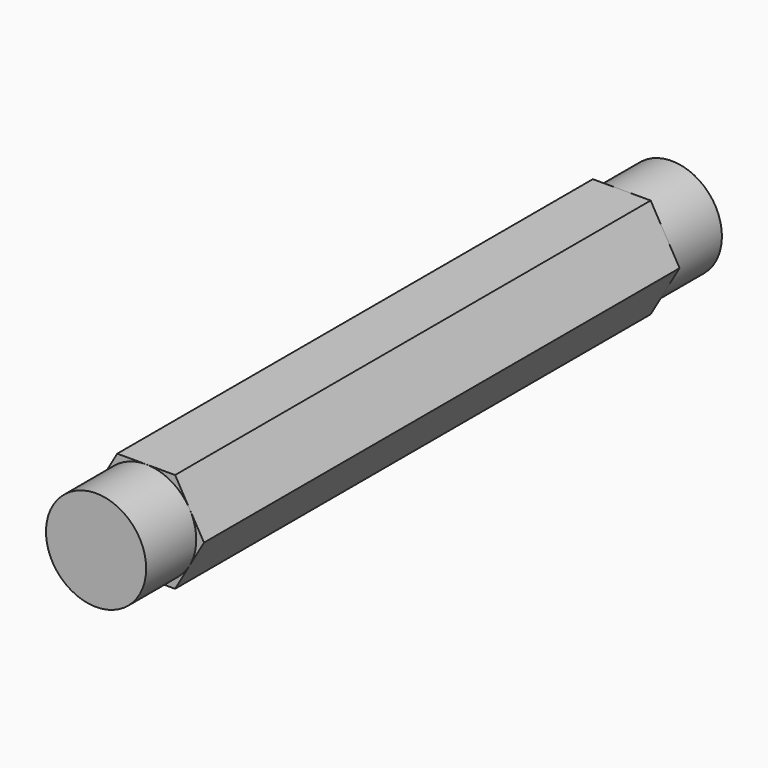
from build123d import *

# Parameters (mm, degrees)
F1_DEPTH = 37.6793125
F2_R     = 6.35
F3_DEPTH = 7.9375


# Not quite as in the source:
# - a pattern or mirror of a feature is missing from the dataset's text; its kind, count and spacing are read off the source's solid


with BuildPart() as f1:
    # F0 (on Front) → F1 (new body, symmetric)
    with BuildSketch(Plane.XZ):
        Polygon((3.6661742094, 6.35), (-3.6661742094, 6.35), (-7.3323484187, 0), (-3.6661742094, -6.35), (3.6661742094, -6.35), (7.3323484187, 0), align=None)
    extrude(amount=F1_DEPTH, both=True)

    # F2 (on face) → F3 (join)
    with BuildSketch(Plane.XZ.offset(37.6793125)):
        Circle(F2_R)
    f3 = extrude(amount=F3_DEPTH)

    # F3_copies: F3 across plane
    add(f3.mirror(Plane.ZX))


solid = f1.part
